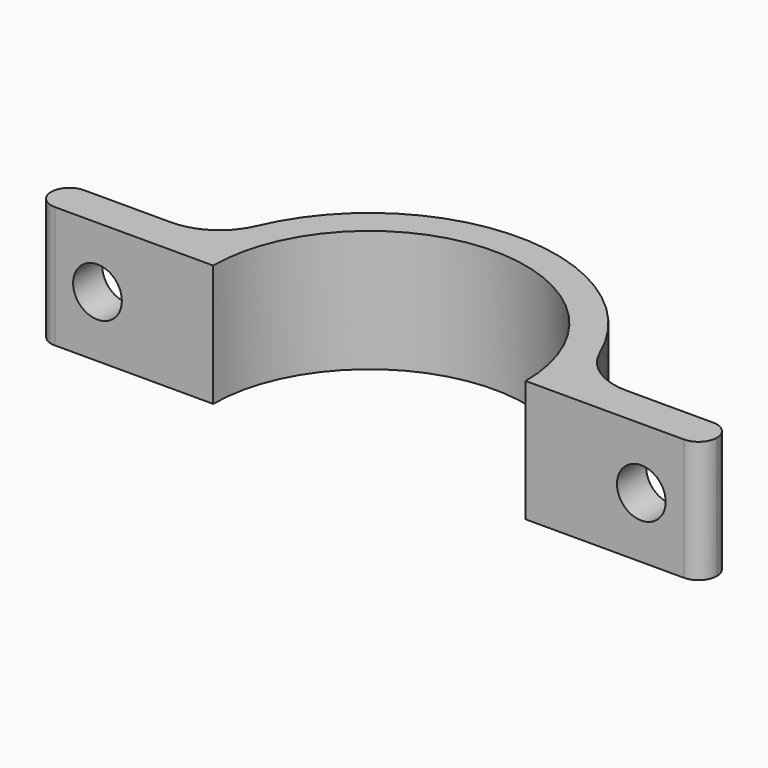
from build123d import *

# Parameters (mm, degrees)
F1_DEPTH = 10
F2_R     = 2
F3_DEPTH = 15.326
F4_R     = 5
F5_R     = 1.49999


# Not quite as in the source:
# - a fillet or chamfer is up to 0.001 mm smaller than in the source, because OpenCascade refuses the exact size


with BuildPart() as f1:
    # F0 (on Top) → F1 (new body)
    with BuildSketch(Plane.XY):
        with BuildLine():
            Line((-15.0284937702, 3), (-27.325, 3))
            Line((-27.325, 3), (-27.325, 0))
            Line((-27.325, 0), (-12.825, 0))
            ThreePointArc((-12.825, 0), (0, 12.825), (12.825, 0))
            Line((12.825, 0), (27.325, 0))
            Line((27.325, 0), (27.325, 3))
            Line((27.325, 3), (15.0284937702, 3))
            ThreePointArc((15.0284937702, 3), (0, 15.325), (-15.0284937702, 3))
        make_face()
    extrude(amount=F1_DEPTH)

    # F2 (on face) → F3 (cut, through all)
    with BuildSketch(Plane.XZ):
        with Locations((-22.325, 5)):
            Circle(F2_R)
        with Locations((22.325, 5)):
            Circle(F2_R)
    extrude(amount=-F3_DEPTH, mode=Mode.SUBTRACT)

    # F4
    f4_edges = [f1.edges().sort_by_distance(p)[0] for p in [
        (-15.028494, 3, 5),
        (15.028494, 3, 5),
    ]]
    fillet(f4_edges, radius=F4_R)

    # F5 (radius 1.5 in the source; OpenCascade refuses exactly that, so slightly less here)
    f5_edges = [f1.edges().sort_by_distance(p)[0] for p in [
        (-27.325, 0, 5),
        (-27.325, 3, 5),
        (27.325, 0, 5),
        (27.325, 3, 5),
    ]]
    fillet(f5_edges, radius=F5_R)


solid = f1.part
